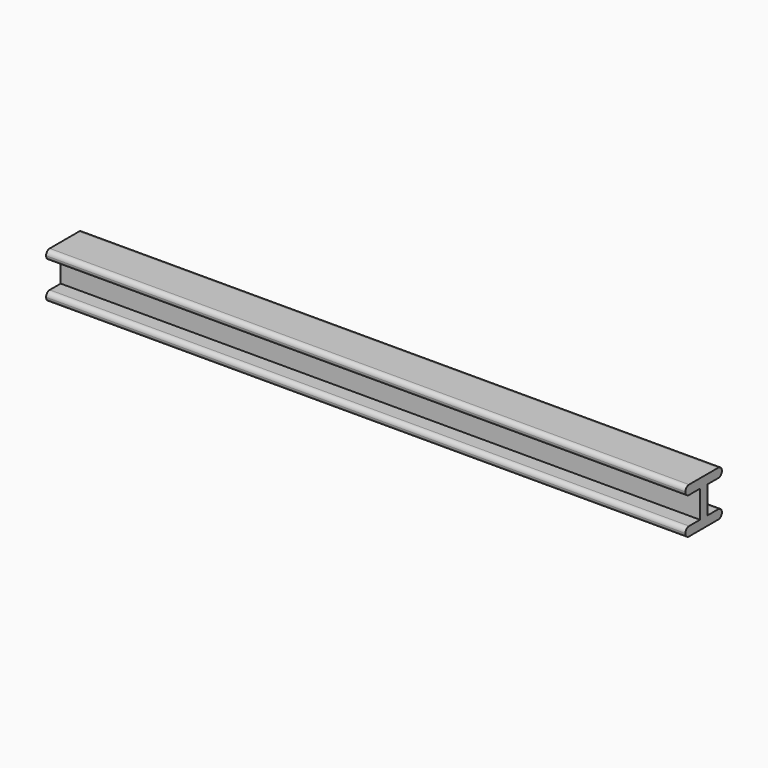
from build123d import *

# Parameters (mm, degrees)
F0_W     = 177.8
F0_H     = 12.7
F1_DEPTH = 12.7
F2_R     = 1.27
F3_W     = 5.08
F3_H     = 7.62
F4_DEPTH = 177.8
F5_R     = 1.26999


# Not quite as in the source:
# - a fillet or chamfer is up to 0.001 mm smaller than in the source, because OpenCascade refuses the exact size


with BuildPart() as f1:
    # F0 (on Top) → F1 (new body)
    with BuildSketch(Plane.XY):
        Rectangle(F0_W, F0_H)
    extrude(amount=F1_DEPTH)

    # F2
    f2_edges = [f1.edges().sort_by_distance(p)[0] for p in [
        (0, 6.35, 0),
        (0, -6.35, 12.7),
        (0, -6.35, 0),
        (0, 6.35, 12.7),
    ]]
    fillet(f2_edges, radius=F2_R)

    # F3 (on face) → F4 (cut)
    with BuildSketch(Plane.YZ.offset(88.9)):
        with Locations((-3.81, 6.35)):
            Rectangle(F3_W, F3_H)
        with Locations((3.81, 6.35)):
            Rectangle(F3_W, F3_H)
    extrude(amount=-F4_DEPTH, mode=Mode.SUBTRACT)

    # F5 (radius 1.27 in the source; OpenCascade refuses exactly that, so slightly less here)
    f5_edges = [f1.edges().sort_by_distance(p)[0] for p in [
        (0, -6.35, 10.16),
        (0, -6.35, 2.54),
        (0, 6.35, 10.16),
        (0, 6.35, 2.54),
    ]]
    fillet(f5_edges, radius=F5_R)


solid = f1.part
